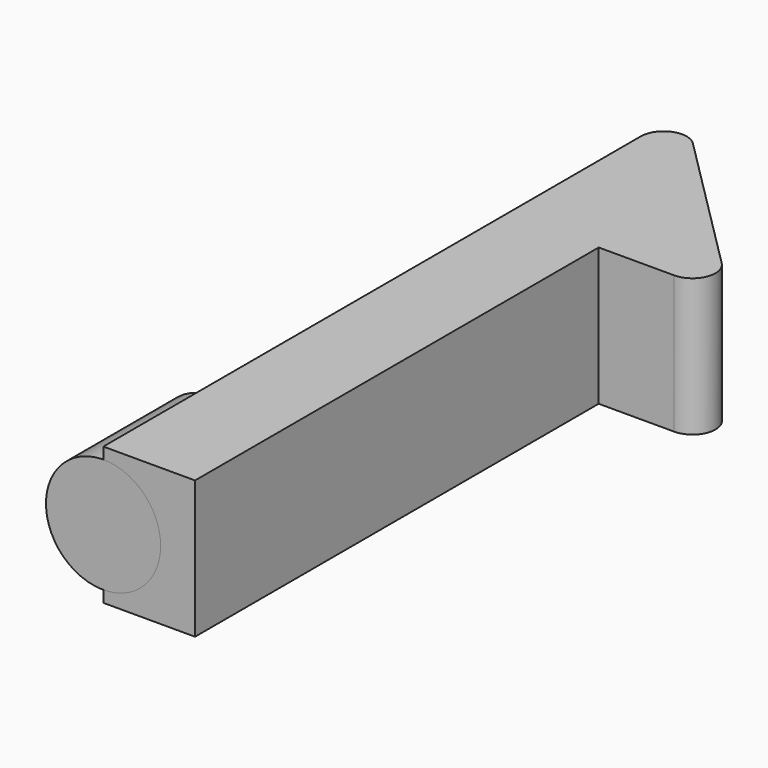
from build123d import *

# Parameters (mm, degrees)
F2_DEPTH = 1.5
F1_R     = 0.6
F3_DEPTH = 5
F1_R_2   = 1.25
F4_DEPTH = 3


with BuildPart() as f2:
    # F0 (on Top) → F2 (new body, symmetric)
    with BuildSketch(Plane.XY):
        with BuildLine():
            Line((0, 11), (0, 0))
            Line((0, 0), (2, 0))
            Line((2, 0), (2, 11))
            Line((2, 11), (3.6464466094, 11))
            ThreePointArc((3.6464466094, 11), (4.1083863757, 11.3086582838), (4, 11.8535533906))
            Line((4, 11.8535533906), (0.8535533906, 15))
            ThreePointArc((0.8535533906, 15), (0.3086582838, 15.1083863757), (0, 14.6464466094))
            Line((0, 14.6464466094), (0, 11))
        make_face()
    extrude(amount=F2_DEPTH, both=True)


with BuildPart() as f3:
    # F1 (on Front) → F3 (new body)
    with BuildSketch(Plane.XZ):
        Circle(F1_R)
    extrude(amount=-F3_DEPTH)

    # F1 (on Front) → F4 (join)
    with BuildSketch(Plane.XZ):
        Circle(F1_R_2)
        Circle(F1_R, mode=Mode.SUBTRACT)
    extrude(amount=-F4_DEPTH)


solid = Compound([f2.part, f3.part])
